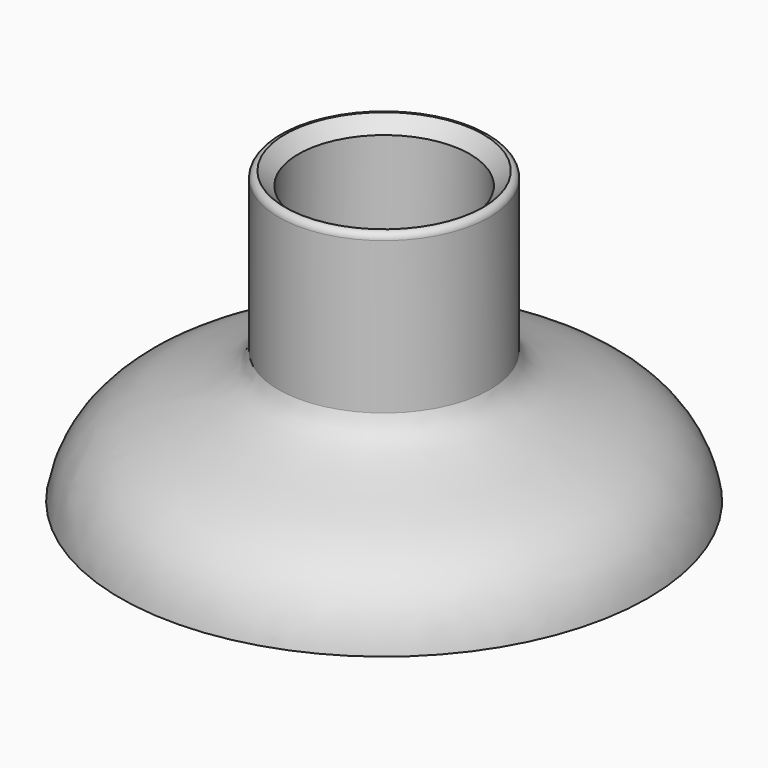
from build123d import *

# Parameters (mm, degrees)
F0_R     = 16
F0_R_2   = 13
F1_DEPTH = 24
F5_R     = 1
F6_SIZE  = 1.99999


# Not quite as in the source:
# - a fillet or chamfer is up to 0.001 mm smaller than in the source, because OpenCascade refuses the exact size


with BuildPart() as f1:
    # F0 (on Top) → F1 (new body)
    with BuildSketch(Plane.XY):
        Circle(F0_R)
        Circle(F0_R_2, mode=Mode.SUBTRACT)
    extrude(amount=F1_DEPTH)


with BuildPart() as f1_1:
    # F2: moved
    add(f1.part.moved(Location((0, 0, 20))))

    # F3 (on Front) → F4 (revolve)
    with BuildSketch(Plane.XZ):
        with BuildLine():
            Line((0, 20), (0, 0))
            Line((0, 0), (40, 0))
            add(Edge.make_bspline(
                [(16, 20), (18.2981714606, 12.3168695718), (37.1231473982, 15.5654279515), (40, 0)],
                knots=[0, 0, 0, 0, 31.2409987036, 31.2409987036, 31.2409987036, 31.2409987036], degree=3))
            Line((16, 20), (0, 20))
        make_face()
    revolve(axis=Axis((0, 0, 10), (0, 0, 1)))

    # F5
    f5_edges = [f1_1.edges().sort_by_distance(p)[0] for p in [
        (-16, 0, 44),
    ]]
    fillet(f5_edges, radius=F5_R)

    # F6 (size 2 in the source; OpenCascade refuses exactly that, so slightly less here)
    f6_edges = [f1_1.edges().sort_by_distance(p)[0] for p in [
        (-13, 0, 44),
    ]]
    chamfer(f6_edges, length=F6_SIZE)


solid = f1_1.part
